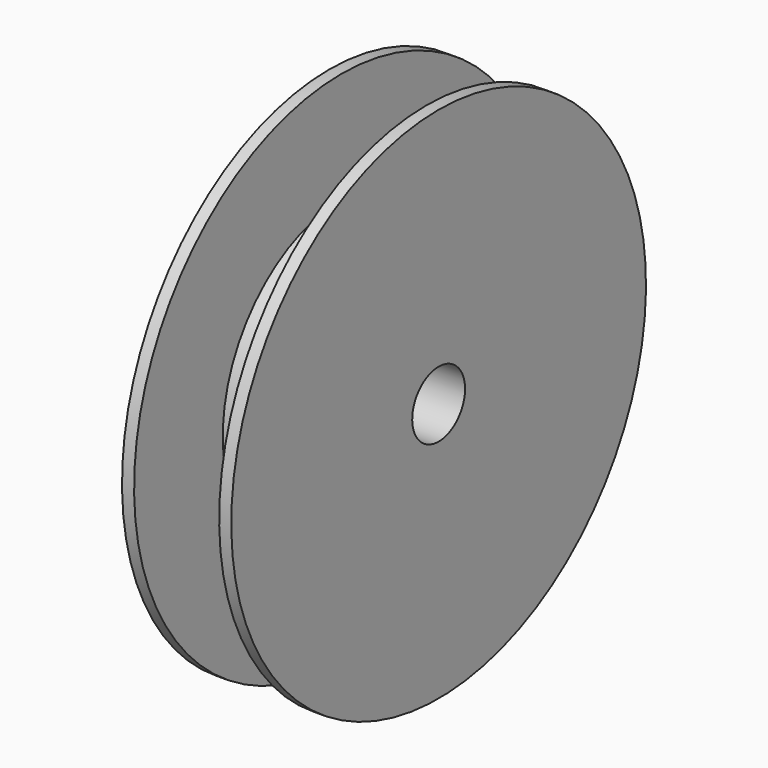
from build123d import *


# Not quite as in the source:
# - the program builds the solid bodies; features that only make, move or delete a surface that nothing else refers to are left out


with BuildPart() as f1:
    # F0 (on Front) → F1 (revolve)
    with BuildSketch(Plane.XZ):
        Polygon((-10.75, 51), (-10.75, 6.5), (0, 6.5), (10.75, 6.5), (10.75, 51), (8.37, 51), (8.37, 29.2), (0, 29.2), (-8.37, 29.2), (-8.37, 51), align=None)
    revolve(axis=Axis((1.0461220518, 0, 0), (1, 0, 0)))


solid = f1.part
